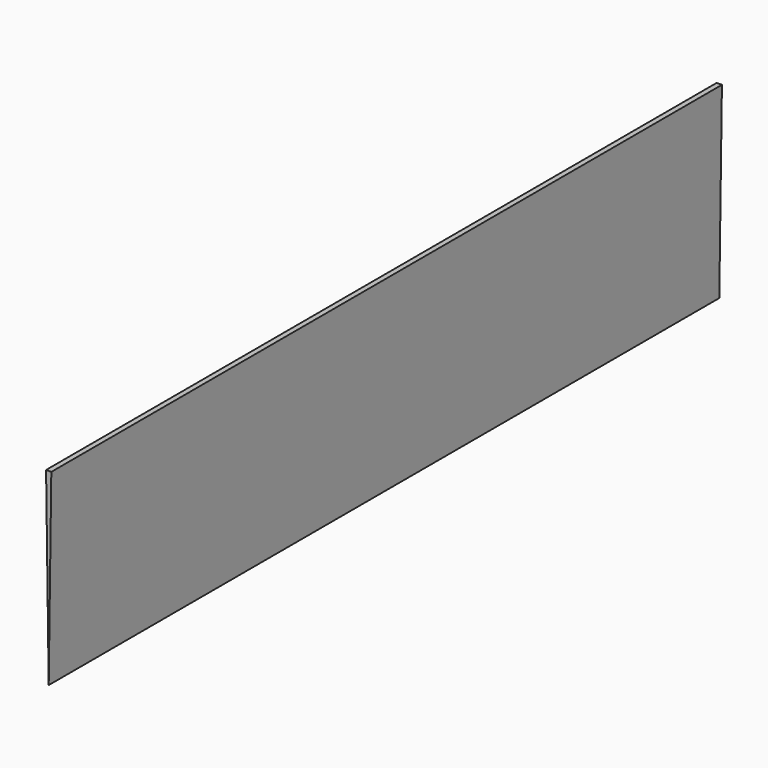
from build123d import *

# Parameters (mm, degrees)
F4_DEPTH = 254


# Not quite as in the source:
# - the program builds the solid bodies; features that only make, move or delete a surface that nothing else refers to are left out


with BuildPart() as f4:
    # F0 (on Front) → F4 (new body, through all)
    with BuildSketch(Plane.XZ):
        Polygon((0.79375, 0), (-0.79375, 0), (0, -57.15), align=None)
    extrude(amount=-F4_DEPTH)


solid = f4.part
